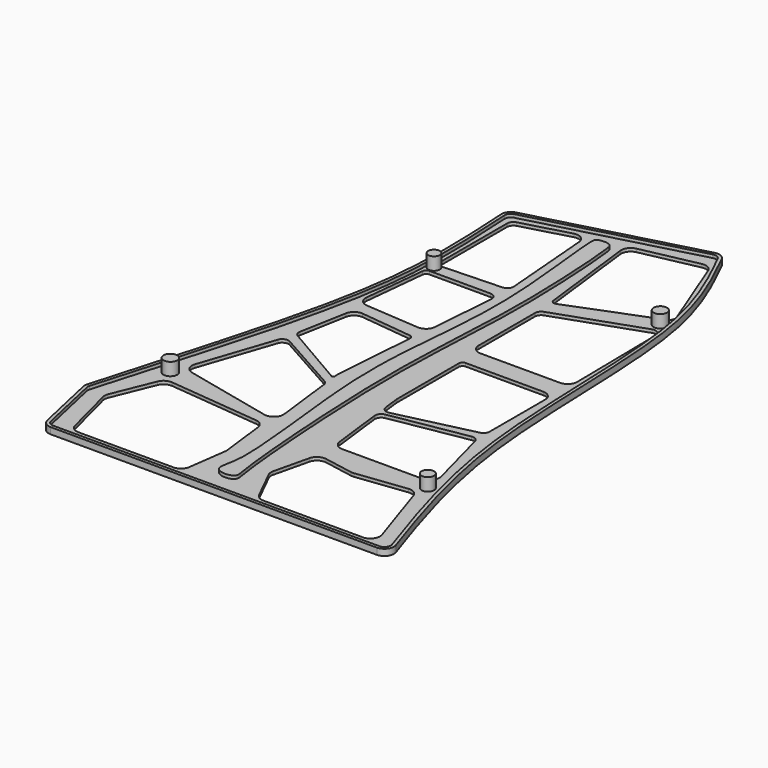
from build123d import *

# Parameters (mm, degrees)
F1_DEPTH = 2
F2_T     = -1
F4_DEPTH = 25
F6_DEPTH = 1
F7_R     = 1.805596873
F7_R_2   = 2.1578935351
F7_R_3   = 1.9765133906
F7_R_4   = 2.1152124275
F8_DEPTH = 4


with BuildPart() as f1:
    # F0 (on Top) → F1 (new body)
    with BuildSketch(Plane.XY):
        with BuildLine():
            Line((-49.4851358235, -62.1426217258), (0, -62.1426217258))
            Line((0, -62.1426217258), (0, 111.8692348227))
            ThreePointArc((0, 111.8692348227), (-1.1461483543, 112.2941981285), (-2.3666764699, 112.2266630973))
            Line((-2.3666764699, 112.2266630973), (-53.9185005165, 98.4881913463))
            ThreePointArc((-53.9185005165, 98.4881913463), (-55.5774706137, 97.3465777746), (-56.140788671, 95.4131517747))
            add(Edge.make_bspline(
                [(-79.0159934188, -38.7652127595), (-75.4066748466, -26.3741188338), (-67.3720925668, 1.3121982666), (-53.8658154229, 51.8521534995), (-55.3337251802, 81.6967592815), (-56.140788671, 95.4131517747)],
                knots=[0.0266747212, 0.0266747212, 0.0266747212, 0.0266747212, 0.32010542, 0.6763464453, 0.9818501019, 0.9818501019, 0.9818501019, 0.9818501019], degree=3))
            ThreePointArc((-79.0159934188, -38.7652127595), (-79.1341073298, -39.5065520197), (-79.0644758325, -40.254005195))
            Line((-79.0644758325, -40.254005195), (-74.7294720781, -59.7924318871))
            ThreePointArc((-74.7294720781, -59.7924318871), (-73.6782671914, -61.4824326673), (-71.8006930229, -62.1426217258))
            Line((-71.8006930229, -62.1426217258), (-49.4851358235, -62.1426217258))
        make_face()
        with BuildLine():
            Line((0, 111.8692348227), (0, -62.1426217258))
            Line((0, -62.1426217258), (30.8165299391, -62.1426217258))
            ThreePointArc((30.8165299391, -62.1426217258), (33.253900074, -60.891686283), (33.6586084163, -58.182106276))
            add(Edge.make_bspline(
                [(1.0925818278, 110.6625662716), (6.0798111199, 100.6235889097), (18.2697213318, 74.8949512389), (14.6415238054, -0.1028802995), (27.5181971714, -40.0131839083), (33.6586084163, -58.182106276)],
                knots=[0.0184672757, 0.0184672757, 0.0184672757, 0.0184672757, 0.2715809047, 0.6516962202, 0.9763935753, 0.9763935753, 0.9763935753, 0.9763935753], degree=3))
            ThreePointArc((1.0925818278, 110.6625662716), (0.6296981306, 111.3414218734), (0, 111.8692348227))
        make_face()
    extrude(amount=F1_DEPTH)

    # F2
    f2_openings = [f1.faces().sort_by_distance(p)[0] for p in [
        (-22.792149, 13.226269, 2),
    ]]
    offset(amount=F2_T, openings=f2_openings, kind=Kind.INTERSECTION)

    # F3 (on face) → F4 (cut)
    with BuildSketch(Plane.XY.offset(1)):
        with BuildLine():
            ThreePointArc((-33.1747278713, 97.4254507718), (-34.447248563, 99.6414089036), (-36.9659150323, 100.0728003371))
            Line((-36.9659150323, 100.0728003371), (-51.6800368392, 95.9955694387))
            ThreePointArc((-51.6800368392, 95.9955694387), (-52.7378441116, 95.2789519405), (-53.1459683276, 94.0681953637))
            Line((-53.1459683276, 94.0681953637), (-53.1459683276, 68.1074285546))
            ThreePointArc((-53.1459683276, 68.1074285546), (-52.534080393, 66.6675865862), (-51.0728234336, 66.108766546))
            Line((-51.0728234336, 66.108766546), (-32.7731894407, 66.7784769741))
            ThreePointArc((-32.7731894407, 66.7784769741), (-31.3512527966, 67.4487071272), (-30.8529447389, 68.9396133474))
            Line((-30.8529447389, 68.9396133474), (-33.1747278713, 97.4254507718))
        make_face()
        with BuildLine():
            ThreePointArc((-52.3045717499, 62.4122569256), (-53.1114939125, 62.1018812925), (-53.502427885, 61.3307606539))
            Line((-53.502427885, 61.3307606539), (-55.5067858477, 41.7504178527))
            ThreePointArc((-55.5067858477, 41.7504178527), (-54.8218801672, 39.5181822921), (-52.7439966222, 38.4531135792))
            Line((-52.7439966222, 38.4531135792), (-35.745224413, 37.1939450636))
            ThreePointArc((-35.745224413, 37.1939450636), (-33.5647904817, 37.9135184161), (-32.5318060601, 39.9641332321))
            Line((-32.5318060601, 39.9641332321), (-31.0280739427, 60.2645135308))
            ThreePointArc((-31.0280739427, 60.2645135308), (-31.557091318, 61.7732332682), (-33.0226094499, 62.4122569256))
            Line((-33.0226094499, 62.4122569256), (-52.3045717499, 62.4122569256))
        make_face()
        with BuildLine():
            ThreePointArc((-19.9998221657, 103.4420753991), (-21.8251398207, 102.2547430379), (-22.3665825474, 100.1456241576))
            Line((-22.3665825474, 100.1456241576), (-18.6234730875, 69.1313126682))
            ThreePointArc((-18.6234730875, 69.1313126682), (-18.0458500202, 68.2420544348), (-16.9890942689, 68.154328181))
            Line((-16.9890942689, 68.154328181), (9.4569612052, 78.507107256))
            ThreePointArc((9.4569612052, 78.507107256), (10.5603268049, 79.5681115462), (10.5902807742, 81.0985521724))
            Line((10.5902807742, 81.0985521724), (1.1209186342, 105.2879292124))
            ThreePointArc((1.1209186342, 105.2879292124), (-0.2444563004, 106.8325636314), (-2.2842811541, 107.1313256883))
            Line((-2.2842811541, 107.1313256883), (-19.9998221657, 103.4420753991))
        make_face()
        with BuildLine():
            ThreePointArc((-16.6849184867, 63.0004316071), (-17.6550600247, 62.2699576447), (-18.023751728, 61.1128780271))
            Line((-18.023751728, 61.1128780271), (-18.023751728, 38.970438419))
            ThreePointArc((-18.023751728, 38.970438419), (-17.1450720716, 36.8491180754), (-15.023751728, 35.970438419))
            Line((-15.023751728, 35.970438419), (9.9982061562, 35.970438419))
            ThreePointArc((9.9982061562, 35.970438419), (12.1346016392, 36.8643011157), (12.9979009704, 39.0132288588))
            Line((12.9979009704, 39.0132288588), (12.5494652265, 70.4494651267))
            ThreePointArc((12.5494652265, 70.4494651267), (11.6950845114, 72.0604571761), (9.8885019251, 72.3084917468))
            Line((9.8885019251, 72.3084917468), (-16.6849184867, 63.0004316071))
        make_face()
        with BuildLine():
            ThreePointArc((-14.6933072247, 29.7106616199), (-15.5447456752, 29.3579842662), (-15.8974230289, 28.5065458156))
            Line((-15.8974230289, 28.5065458156), (-15.8974230289, 4.2735014143))
            ThreePointArc((-15.8974230289, 4.2735014143), (-15.8920148557, 4.0934464473), (-15.8758098348, 3.9140406592))
            Line((-15.8758098348, 3.9140406592), (-15.2843265093, -0.9868173831))
            ThreePointArc((-15.2843265093, -0.9868173831), (-14.4442900555, -2.3865988249), (-12.8410136224, -2.6940951782))
            Line((-12.8410136224, -2.6940951782), (11.1916682373, 2.9560030287))
            ThreePointArc((11.1916682373, 2.9560030287), (12.3016587993, 3.6610363417), (12.7339465544, 4.9029213272))
            Line((12.7339465544, 4.9029213272), (12.7339465544, 26.7106616199))
            ThreePointArc((12.7339465544, 26.7106616199), (11.8552668979, 28.8319819635), (9.7339465544, 29.7106616199))
            Line((9.7339465544, 29.7106616199), (-13.4863620624, 29.7106616199))
            Line((-13.4863620624, 29.7106616199), (-14.6933072247, 29.7106616199))
        make_face()
        with BuildLine():
            ThreePointArc((-12.7038883673, -22.3675739897), (-11.7156796607, -24.2529275103), (-9.7255015614, -25.0081132345))
            Line((-9.7255015614, -25.0081132345), (15.4653231801, -25.0081132345))
            ThreePointArc((15.4653231801, -25.0081132345), (17.8429782142, -23.8375274956), (18.365133865, -21.2392842602))
            Line((18.365133865, -21.2392842602), (13.1038161615, -1.3950460695))
            ThreePointArc((13.1038161615, -1.3950460695), (12.2508434616, -0.2244191117), (10.8313067374, 0.0634096394))
            Line((10.8313067374, 0.0634096394), (-13.0028014186, -4.0395499957))
            ThreePointArc((-13.0028014186, -4.0395499957), (-14.2675641257, -4.8159975769), (-14.6490903218, -6.2501988575))
            Line((-14.6490903218, -6.2501988575), (-12.7038883673, -22.3675739897))
        make_face()
        with BuildLine():
            Line((-35.4512886795, 5.3128479066), (-33.5536682044, 31.3127004157))
            ThreePointArc((-33.5536682044, 31.3127004157), (-33.8277963369, 32.1690827431), (-34.618752707, 32.596780001))
            Line((-34.618752707, 32.596780001), (-50.8797757491, 34.4429797578))
            ThreePointArc((-50.8797757491, 34.4429797578), (-53.0042889334, 33.8725062121), (-54.1684863022, 32.0060548137))
            Line((-54.1684863022, 32.0060548137), (-56.880903372, 17.2937456147))
            ThreePointArc((-56.880903372, 17.2937456147), (-56.7310323407, 16.0953195392), (-55.9185597229, 15.2016895096))
            Line((-55.9185597229, 15.2016895096), (-36.1170125467, 3.7003735849))
            ThreePointArc((-36.1170125467, 3.7003735849), (-35.5804548922, 3.7154404772), (-35.3546596398, 4.2024082706))
            Line((-35.3546596398, 4.2024082706), (-35.4421856248, 4.9276230132))
            ThreePointArc((-35.4421856248, 4.9276230132), (-35.4560362544, 5.1200157175), (-35.4512886795, 5.3128479066))
        make_face()
        with BuildLine():
            Line((-64.0395783428, -16.2671541998), (-36.1582523419, -22.6404937465))
            ThreePointArc((-36.1582523419, -22.6404937465), (-33.4822265493, -21.9452613575), (-32.5113447747, -19.3564680679))
            Line((-32.5113447747, -19.3564680679), (-34.7259230115, -1.0071197549))
            ThreePointArc((-34.7259230115, -1.0071197549), (-35.0490889427, -0.1348509938), (-35.7318744538, 0.4968870504))
            Line((-35.7318744538, 0.4968870504), (-55.6239252799, 11.6729109131))
            ThreePointArc((-55.6239252799, 11.6729109131), (-57.3217994375, 11.7958485481), (-58.4993324698, 10.5664965743))
            Line((-58.4993324698, 10.5664965743), (-66.2147087239, -12.3867398214))
            ThreePointArc((-66.2147087239, -12.3867398214), (-65.9879721402, -14.8094765224), (-64.0395783428, -16.2671541998))
        make_face()
        with BuildLine():
            Line((-31.4659024534, -43.1040638044), (-33.1815712106, -28.8885336905))
            ThreePointArc((-33.1815712106, -28.8885336905), (-34.0599886763, -27.1055358648), (-35.8602223312, -26.2630055815))
            Line((-35.8602223312, -26.2630055815), (-64.5866806463, -23.3784572425))
            ThreePointArc((-64.5866806463, -23.3784572425), (-66.4348312228, -23.7939303302), (-67.6656324914, -25.2338632026))
            Line((-67.6656324914, -25.2338632026), (-72.9054536357, -38.1258745342))
            ThreePointArc((-72.9054536357, -38.1258745342), (-73.1195676129, -39.0555207205), (-73.0309937761, -40.0053846592))
            Line((-73.0309937761, -40.0053846592), (-68.8365169234, -56.2522053151))
            ThreePointArc((-68.8365169234, -56.2522053151), (-67.768907642, -57.8739633244), (-65.9317606232, -58.5022780942))
            Line((-65.9317606232, -58.5022780942), (-36.0877538217, -58.5022780942))
            ThreePointArc((-36.0877538217, -58.5022780942), (-34.1151083479, -57.7625147709), (-33.1153233884, -55.9080579839))
            Line((-33.1153233884, -55.9080579839), (-31.471858826, -43.8693044493))
            ThreePointArc((-31.471858826, -43.8693044493), (-31.4443801332, -43.4868748305), (-31.4659024534, -43.1040638044))
        make_face()
        with BuildLine():
            ThreePointArc((-9.5868923333, -31.5545818373), (-11.7643199031, -31.9965384312), (-13.0405377373, -33.8152699927))
            Line((-13.0405377373, -33.8152699927), (-15.6481497381, -44.8263009438))
            ThreePointArc((-15.6481497381, -44.8263009438), (-15.7095820499, -45.8574778896), (-15.4176040785, -46.8483606711))
            Line((-15.4176040785, -46.8483606711), (-10.4758925707, -56.8330048818))
            ThreePointArc((-10.4758925707, -56.8330048818), (-9.3695564272, -58.0510209571), (-7.7871816869, -58.5022780942))
            Line((-7.7871816869, -58.5022780942), (23.5132491834, -58.5022780942))
            ThreePointArc((23.5132491834, -58.5022780942), (25.945204351, -57.2588640052), (26.3612079724, -54.5593408026))
            Line((26.3612079724, -54.5593408026), (19.3480585919, -33.3774864033))
            ThreePointArc((19.3480585919, -33.3774864033), (18.1075572043, -31.7874253328), (16.1406390477, -31.342036889))
            Line((16.1406390477, -31.342036889), (0.448911769, -33.235867511))
            ThreePointArc((0.448911769, -33.235867511), (0.0009990597, -33.2561764636), (-0.4449378467, -33.2095018002))
            Line((-0.4449378467, -33.2095018002), (-9.5868923333, -31.5545818373))
        make_face()
    extrude(amount=-F4_DEPTH, mode=Mode.SUBTRACT)

    # F5 (on face) → F6 (join)
    with BuildSketch(Plane.XY.offset(1)):
        with BuildLine():
            add(Edge.make_bspline(
                [(-24.458264932, 97.4254507718), (-24.6551575661, 98.7633328982), (-25.0467132646, 99.9930667353), (-29.5789047362, 100.0350380868), (-30.2029089384, 96.5639961489), (-25.4422809247, 62.9335898587), (-28.1072891429, 33.3352921574), (-30.8522295498, 1.8892451859), (-23.1029838696, -45.2019458341), (-26.9136456134, -53.0130745697), (-23.9662275582, -55.0350740432), (-19.4114381211, -54.4331476398), (-21.2743532793, -48.0203192629), (-24.8823302963, 0.5592596332), (-23.910287767, 32.8904719172), (-21.92099784, 63.3359096043), (-23.7566593864, 92.6580529265), (-24.458264932, 97.4254507718)],
                knots=[0, 0, 0, 0, 0.0257827129, 0.0559780929, 0.080977294, 0.1736530027, 0.265656082, 0.3604260352, 0.4720552125, 0.513992159, 0.5402401983, 0.5703296774, 0.6051962704, 0.7181074238, 0.8150213738, 0.908126099, 1, 1, 1, 1], degree=3))
        make_face()
    extrude(amount=F6_DEPTH)

    # F7 (on face) → F8 (join)
    with BuildSketch(Plane.XY.offset(1)):
        with Locations((-52.534080393, 64.5554438233)):
            Circle(F7_R)
        with Locations((-68.2824328542, -19.4576382637)):
            Circle(F7_R_2)
        with Locations((19.5783078671, -28.0128829181)):
            Circle(F7_R_3)
        with Locations((9.8885019251, 75.5478069186)):
            Circle(F7_R_4)
    extrude(amount=F8_DEPTH)


solid = f1.part
